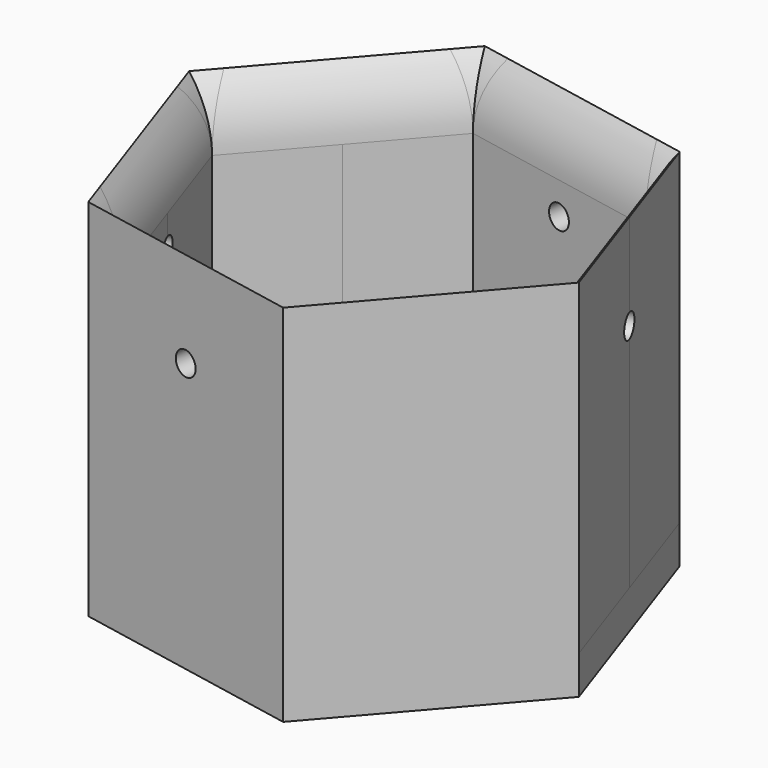
from build123d import *

# Parameters (mm, degrees)
F1_DEPTH      = 2.032
F3_DEPTH      = 19.05
F4_T4_DEPTH   = 36.3985226281
F4_T10_DEPTH  = 36.3985226281
F4_T16_DEPTH  = 36.3985226281
F4_T22_DEPTH  = 36.3985226281
F4_T28_DEPTH  = 36.3985226281
F4_T34_DEPTH  = 36.3985226281
F4_T41_DEPTH  = 36.3985226281
F4_T47_DEPTH  = 36.3985226281
F4_T56_DEPTH  = 36.3985226281
F4_T62_DEPTH  = 36.3985226281
F4_T71_DEPTH  = 36.3985226281
F4_T77_DEPTH  = 36.3985226281
F4_T86_DEPTH  = 36.3985226281
F4_T92_DEPTH  = 36.3985226281
F4_T101_DEPTH = 36.3985226281
F4_T107_DEPTH = 36.3985226281
F4_T116_DEPTH = 36.3985226281
F4_T122_DEPTH = 36.3985226281
F6_R          = 0.635
F7_DEPTH      = 25.4
F5_R          = 0.635
F8_DEPTH      = 25.4


# Not quite as in the source:
# - a fillet or chamfer that OpenCascade refuses, or shapes differently, is made with other operations: its cross-section is extruded or revolved along the edge and cut away or added


with BuildPart() as f1:
    # F0 (on Top) → F1 (new body)
    with BuildSketch(Plane.XY):
        Polygon((-123.0130245504, 41.1086249019), (-114.844562537, 50.5241579017), (-118.9144222983, 62.306020015), (-131.1527440729, 64.6723491286), (-139.3212060863, 55.2568161288), (-135.2513463251, 43.4749540155), align=None)
    extrude(amount=F1_DEPTH)

    # F2 (on face) → F3 (join)
    with BuildSketch(Plane.XY.offset(2.032)):
        Polygon((-131.1527440729, 64.6723491286), (-135.2369750796, 59.9645826287), (-134.2776702834, 59.1323360859), (-130.6739370422, 63.2862477035), (-119.8754178293, 61.1983102503), (-118.079891464, 56.0004299062), (-116.8794924177, 56.4150889583), (-118.9144222983, 62.306020015), align=None)
        Polygon((-134.2776702834, 59.1323360859), (-135.2369750796, 59.9645826287), (-139.3212060863, 55.2568161288), (-137.2862762057, 49.3658850722), (-136.0858771593, 49.7805441243), (-137.8814035246, 54.9784244684), align=None)
        Polygon((-136.0858771593, 49.7805441243), (-137.2862762057, 49.3658850722), (-135.2513463251, 43.4749540155), (-123.0130245504, 41.1086249019), (-118.9287935437, 45.8163914018), (-119.88809834, 46.6486379446), (-123.4918315812, 42.494726327), (-134.2903507941, 44.5826637802), align=None)
        Polygon((-116.2843650988, 50.8025495621), (-119.88809834, 46.6486379446), (-118.9287935437, 45.8163914018), (-114.844562537, 50.5241579017), (-116.8794924177, 56.4150889583), (-118.079891464, 56.0004299062), align=None)
    extrude(amount=F3_DEPTH)

    # F4: fillet of radius 5.08 on 6 edges, made by hand


with BuildPart() as f4_tool2:
    # F4_s3 → F4_t4 (new body)
    with BuildSketch(Plane(origin=(-40.3193780899, -46.4748975157, 0), x_dir=(0, 0, 1), z_dir=(0.6553122384, 0.7553581073, 0))):
        with BuildLine():
            ThreePointArc((21.082, -145.2578703952), (19.5941024484, -141.6657679468), (16.002, -140.1778703952))
            Line((16.002, -140.1778703952), (21.082, -140.1778703952))
            Line((21.082, -140.1778703952), (21.082, -145.2578703952))
        make_face()
    extrude(amount=F4_T4_DEPTH)

    split(bisect_by=Plane(origin=(7.0863744403, 36.6497331747, 0), x_dir=(0, 0, 1), z_dir=(-0.1898379922, -0.981815429, 0)), keep=Keep.TOP)

    split(bisect_by=Plane(origin=(-106.215781989, -36.6905785323, 0), x_dir=(0, 0, 1), z_dir=(0.9451960995, 0.3265031907, 0)), keep=Keep.TOP)


with BuildPart() as f1_1:
    add(f1.part)

    # F4_t1: cut F4_tool2
    add(f4_tool2.part, mode=Mode.SUBTRACT)


with BuildPart() as f4_tool8:
    # F4_s9 → F4_t10 (new body)
    with BuildSketch(Plane(origin=(-150.2293674314, 29.0474570301, 0), x_dir=(0, 0, 1), z_dir=(0.981815429, -0.1898379922, 0))):
        with BuildLine():
            ThreePointArc((21.082, -42.4085365971), (19.5941024484, -38.8164341487), (16.002, -37.3285365971))
            Line((16.002, -37.3285365971), (21.082, -37.3285365971))
            Line((21.082, -37.3285365971), (21.082, -42.4085365971))
        make_face()
    extrude(amount=F4_T10_DEPTH)

    split(bisect_by=Plane(origin=(-88.2097962936, -30.4706927504, 0), x_dir=(0, 0, 1), z_dir=(-0.9451960995, -0.3265031907, 0)), keep=Keep.TOP)

    split(bisect_by=Plane(origin=(-105.8844908623, 91.8602740219, 0), x_dir=(0, 0, 1), z_dir=(0.7553581073, -0.6553122384, 0)), keep=Keep.TOP)


with BuildPart() as f1_2:
    add(f1_1.part)

    # F4_t7: cut F4_tool8
    add(f4_tool8.part, mode=Mode.SUBTRACT)


with BuildPart() as f4_tool14:
    # F4_s15 → F4_t16 (new body)
    with BuildSketch(Plane(origin=(-35.8122120569, 103.6729934642, 0), x_dir=(0, 0, 1), z_dir=(0.3265031907, -0.9451960995, 0))):
        with BuildLine():
            ThreePointArc((21.082, 88.2443337981), (19.5941024484, 91.8364362465), (16.002, 93.3243337981))
            Line((16.002, 93.3243337981), (21.082, 93.3243337981))
            Line((21.082, 93.3243337981), (21.082, 88.2443337981))
        make_face()
    extrude(amount=F4_T16_DEPTH)

    split(bisect_by=Plane(origin=(-91.4949189189, 79.3765758805, 0), x_dir=(0, 0, 1), z_dir=(-0.7553581073, 0.6553122384, 0)), keep=Keep.TOP)

    split(bisect_by=Plane(origin=(7.0863744403, 36.6497331747, 0), x_dir=(0, 0, 1), z_dir=(-0.1898379922, -0.981815429, 0)), keep=Keep.TOP)


with BuildPart() as f1_3:
    add(f1_2.part)

    # F4_t13: cut F4_tool14
    add(f4_tool14.part, mode=Mode.SUBTRACT)


with BuildPart() as f4_tool20:
    # F4_s21 → F4_t22 (new body)
    with BuildSketch(Plane(origin=(-16.4669807523, -18.9809783561, 0), x_dir=(0, 0, 1), z_dir=(-0.6553122384, -0.7553581073, 0))):
        with BuildLine():
            ThreePointArc((21.082, 116.0478703952), (19.5941024484, 119.6399728436), (16.002, 121.1278703952))
            Line((16.002, 121.1278703952), (21.082, 121.1278703952))
            Line((21.082, 121.1278703952), (21.082, 116.0478703952))
        make_face()
    extrude(amount=F4_T22_DEPTH)

    split(bisect_by=Plane(origin=(-88.2097962936, -30.4706927504, 0), x_dir=(0, 0, 1), z_dir=(-0.9451960995, -0.3265031907, 0)), keep=Keep.TOP)

    split(bisect_by=Plane(origin=(3.4699606884, 17.9461492514, 0), x_dir=(0, 0, 1), z_dir=(0.1898379922, 0.981815429, 0)), keep=Keep.TOP)


with BuildPart() as f1_4:
    add(f1_3.part)

    # F4_t19: cut F4_tool20
    add(f4_tool20.part, mode=Mode.SUBTRACT)


with BuildPart() as f4_tool26:
    # F4_s27 → F4_t28 (new body)
    with BuildSketch(Plane(origin=(-114.4927363208, 22.1376345743, 0), x_dir=(0, 0, 1), z_dir=(-0.981815429, 0.1898379922, 0))):
        with BuildLine():
            ThreePointArc((21.082, 13.1985365971), (19.5941024484, 16.7906390456), (16.002, 18.2785365971))
            Line((16.002, 18.2785365971), (21.082, 18.2785365971))
            Line((21.082, 18.2785365971), (21.082, 13.1985365971))
        make_face()
    extrude(amount=F4_T28_DEPTH)

    split(bisect_by=Plane(origin=(-91.4949189189, 79.3765758805, 0), x_dir=(0, 0, 1), z_dir=(-0.7553581073, 0.6553122384, 0)), keep=Keep.TOP)

    split(bisect_by=Plane(origin=(-106.215781989, -36.6905785323, 0), x_dir=(0, 0, 1), z_dir=(0.9451960995, 0.3265031907, 0)), keep=Keep.TOP)


with BuildPart() as f1_5:
    add(f1_4.part)

    # F4_t25: cut F4_tool26
    add(f4_tool26.part, mode=Mode.SUBTRACT)


with BuildPart() as f4_tool32:
    # F4_s33 → F4_t34 (new body)
    with BuildSketch(Plane(origin=(-23.9279782839, 69.2692518489, 0), x_dir=(0, 0, 1), z_dir=(-0.3265031907, 0.9451960995, 0))):
        with BuildLine():
            ThreePointArc((21.082, -117.4543337981), (19.5941024484, -113.8622313496), (16.002, -112.3743337981))
            Line((16.002, -112.3743337981), (21.082, -112.3743337981))
            Line((21.082, -112.3743337981), (21.082, -117.4543337981))
        make_face()
    extrude(amount=F4_T34_DEPTH)

    split(bisect_by=Plane(origin=(-105.8844908623, 91.8602740219, 0), x_dir=(0, 0, 1), z_dir=(0.7553581073, -0.6553122384, 0)), keep=Keep.TOP)

    split(bisect_by=Plane(origin=(3.4699606884, 17.9461492514, 0), x_dir=(0, 0, 1), z_dir=(0.1898379922, 0.981815429, 0)), keep=Keep.TOP)


with BuildPart() as f1_6:
    add(f1_5.part)

    # F4_t31: cut F4_tool32
    add(f4_tool32.part, mode=Mode.SUBTRACT)


with BuildPart() as f4_tool39:
    # F4_s40 → F4_t41 (new body)
    with BuildSketch(Plane(origin=(-23.9279782839, 69.2692518489, 0), x_dir=(0, 0, 1), z_dir=(-0.3265031907, 0.9451960995, 0))):
        with BuildLine():
            ThreePointArc((21.082, -117.4543337981), (19.5941024484, -113.8622313496), (16.002, -112.3743337981))
            Line((16.002, -112.3743337981), (21.082, -112.3743337981))
            Line((21.082, -112.3743337981), (21.082, -117.4543337981))
        make_face()
    extrude(amount=F4_T41_DEPTH)

    split(bisect_by=Plane(origin=(-106.8437956585, 92.6925205646, 0), x_dir=(0, 0, 1), z_dir=(0.7553581073, -0.6553122384, 0)), keep=Keep.TOP)

    split(bisect_by=Plane(origin=(-105.8844908623, 91.8602740219, 0), x_dir=(0, 0, 1), z_dir=(-0.7553581073, 0.6553122384, 0)), keep=Keep.TOP)

    split(bisect_by=Plane(origin=(-107.4161810353, -37.1052375844, 0), x_dir=(0, 0, 1), z_dir=(0.9451960995, 0.3265031907, 0)), keep=Keep.TOP)


with BuildPart() as f4_tool45:
    # F4_s46 → F4_t47 (new body)
    with BuildSketch(Plane(origin=(-40.3193780899, -46.4748975157, 0), x_dir=(0, 0, 1), z_dir=(0.6553122384, 0.7553581073, 0))):
        with BuildLine():
            ThreePointArc((21.082, -145.2578703952), (19.5941024484, -141.6657679468), (16.002, -140.1778703952))
            Line((16.002, -140.1778703952), (21.082, -140.1778703952))
            Line((21.082, -140.1778703952), (21.082, -145.2578703952))
        make_face()
    extrude(amount=F4_T47_DEPTH)

    split(bisect_by=Plane(origin=(-106.8437956585, 92.6925205646, 0), x_dir=(0, 0, 1), z_dir=(0.7553581073, -0.6553122384, 0)), keep=Keep.TOP)

    split(bisect_by=Plane(origin=(-106.215781989, -36.6905785323, 0), x_dir=(0, 0, 1), z_dir=(-0.9451960995, -0.3265031907, 0)), keep=Keep.TOP)

    split(bisect_by=Plane(origin=(-107.4161810353, -37.1052375844, 0), x_dir=(0, 0, 1), z_dir=(0.9451960995, 0.3265031907, 0)), keep=Keep.TOP)


with BuildPart() as f4_tool39_1:
    add(f4_tool39.part)

    # F4_t51: intersect F4_tool45
    add(f4_tool45.part, mode=Mode.INTERSECT)


with BuildPart() as f1_7:
    add(f1_6.part)

    # F4_t37: cut F4_tool39
    add(f4_tool39_1.part, mode=Mode.SUBTRACT)


with BuildPart() as f4_tool54:
    # F4_s55 → F4_t56 (new body)
    with BuildSketch(Plane(origin=(-40.3193780899, -46.4748975157, 0), x_dir=(0, 0, 1), z_dir=(0.6553122384, 0.7553581073, 0))):
        with BuildLine():
            ThreePointArc((21.082, -145.2578703952), (19.5941024484, -141.6657679468), (16.002, -140.1778703952))
            Line((16.002, -140.1778703952), (21.082, -140.1778703952))
            Line((21.082, -140.1778703952), (21.082, -145.2578703952))
        make_face()
    extrude(amount=F4_T56_DEPTH)

    split(bisect_by=Plane(origin=(-106.8437956585, 92.6925205646, 0), x_dir=(0, 0, 1), z_dir=(0.7553581073, -0.6553122384, 0)), keep=Keep.TOP)

    split(bisect_by=Plane(origin=(7.3274686905, 37.8966387696, 0), x_dir=(0, 0, 1), z_dir=(-0.1898379922, -0.981815429, 0)), keep=Keep.TOP)

    split(bisect_by=Plane(origin=(7.0863744403, 36.6497331747, 0), x_dir=(0, 0, 1), z_dir=(0.1898379922, 0.981815429, 0)), keep=Keep.TOP)


with BuildPart() as f4_tool60:
    # F4_s61 → F4_t62 (new body)
    with BuildSketch(Plane(origin=(-150.2293674314, 29.0474570301, 0), x_dir=(0, 0, 1), z_dir=(0.981815429, -0.1898379922, 0))):
        with BuildLine():
            ThreePointArc((21.082, -42.4085365971), (19.5941024484, -38.8164341487), (16.002, -37.3285365971))
            Line((16.002, -37.3285365971), (21.082, -37.3285365971))
            Line((21.082, -37.3285365971), (21.082, -42.4085365971))
        make_face()
    extrude(amount=F4_T62_DEPTH)

    split(bisect_by=Plane(origin=(-106.8437956585, 92.6925205646, 0), x_dir=(0, 0, 1), z_dir=(0.7553581073, -0.6553122384, 0)), keep=Keep.TOP)

    split(bisect_by=Plane(origin=(7.3274686905, 37.8966387696, 0), x_dir=(0, 0, 1), z_dir=(-0.1898379922, -0.981815429, 0)), keep=Keep.TOP)

    split(bisect_by=Plane(origin=(-105.8844908623, 91.8602740219, 0), x_dir=(0, 0, 1), z_dir=(-0.7553581073, 0.6553122384, 0)), keep=Keep.TOP)


with BuildPart() as f4_tool54_1:
    add(f4_tool54.part)

    # F4_t66: intersect F4_tool60
    add(f4_tool60.part, mode=Mode.INTERSECT)


with BuildPart() as f1_8:
    add(f1_7.part)

    # F4_t52: cut F4_tool54
    add(f4_tool54_1.part, mode=Mode.SUBTRACT)


with BuildPart() as f4_tool69:
    # F4_s70 → F4_t71 (new body)
    with BuildSketch(Plane(origin=(-150.2293674314, 29.0474570301, 0), x_dir=(0, 0, 1), z_dir=(0.981815429, -0.1898379922, 0))):
        with BuildLine():
            ThreePointArc((21.082, -42.4085365971), (19.5941024484, -38.8164341487), (16.002, -37.3285365971))
            Line((16.002, -37.3285365971), (21.082, -37.3285365971))
            Line((21.082, -37.3285365971), (21.082, -42.4085365971))
        make_face()
    extrude(amount=F4_T71_DEPTH)

    split(bisect_by=Plane(origin=(7.3274686905, 37.8966387696, 0), x_dir=(0, 0, 1), z_dir=(-0.1898379922, -0.981815429, 0)), keep=Keep.TOP)

    split(bisect_by=Plane(origin=(-87.0093972473, -30.0560336983, 0), x_dir=(0, 0, 1), z_dir=(-0.9451960995, -0.3265031907, 0)), keep=Keep.TOP)

    split(bisect_by=Plane(origin=(-88.2097962936, -30.4706927504, 0), x_dir=(0, 0, 1), z_dir=(0.9451960995, 0.3265031907, 0)), keep=Keep.TOP)


with BuildPart() as f4_tool75:
    # F4_s76 → F4_t77 (new body)
    with BuildSketch(Plane(origin=(-35.8122120569, 103.6729934642, 0), x_dir=(0, 0, 1), z_dir=(0.3265031907, -0.9451960995, 0))):
        with BuildLine():
            ThreePointArc((21.082, 88.2443337981), (19.5941024484, 91.8364362465), (16.002, 93.3243337981))
            Line((16.002, 93.3243337981), (21.082, 93.3243337981))
            Line((21.082, 93.3243337981), (21.082, 88.2443337981))
        make_face()
    extrude(amount=F4_T77_DEPTH)

    split(bisect_by=Plane(origin=(7.3274686905, 37.8966387696, 0), x_dir=(0, 0, 1), z_dir=(-0.1898379922, -0.981815429, 0)), keep=Keep.TOP)

    split(bisect_by=Plane(origin=(-87.0093972473, -30.0560336983, 0), x_dir=(0, 0, 1), z_dir=(-0.9451960995, -0.3265031907, 0)), keep=Keep.TOP)

    split(bisect_by=Plane(origin=(7.0863744403, 36.6497331747, 0), x_dir=(0, 0, 1), z_dir=(0.1898379922, 0.981815429, 0)), keep=Keep.TOP)


with BuildPart() as f4_tool69_1:
    add(f4_tool69.part)

    # F4_t81: intersect F4_tool75
    add(f4_tool75.part, mode=Mode.INTERSECT)


with BuildPart() as f1_9:
    add(f1_8.part)

    # F4_t67: cut F4_tool69
    add(f4_tool69_1.part, mode=Mode.SUBTRACT)


with BuildPart() as f4_tool84:
    # F4_s85 → F4_t86 (new body)
    with BuildSketch(Plane(origin=(-35.8122120569, 103.6729934642, 0), x_dir=(0, 0, 1), z_dir=(0.3265031907, -0.9451960995, 0))):
        with BuildLine():
            ThreePointArc((21.082, 88.2443337981), (19.5941024484, 91.8364362465), (16.002, 93.3243337981))
            Line((16.002, 93.3243337981), (21.082, 93.3243337981))
            Line((21.082, 93.3243337981), (21.082, 88.2443337981))
        make_face()
    extrude(amount=F4_T86_DEPTH)

    split(bisect_by=Plane(origin=(-87.0093972473, -30.0560336983, 0), x_dir=(0, 0, 1), z_dir=(-0.9451960995, -0.3265031907, 0)), keep=Keep.TOP)

    split(bisect_by=Plane(origin=(-90.5356141227, 78.5443293377, 0), x_dir=(0, 0, 1), z_dir=(-0.7553581073, 0.6553122384, 0)), keep=Keep.TOP)

    split(bisect_by=Plane(origin=(-91.4949189189, 79.3765758805, 0), x_dir=(0, 0, 1), z_dir=(0.7553581073, -0.6553122384, 0)), keep=Keep.TOP)


with BuildPart() as f4_tool90:
    # F4_s91 → F4_t92 (new body)
    with BuildSketch(Plane(origin=(-16.4669807523, -18.9809783561, 0), x_dir=(0, 0, 1), z_dir=(-0.6553122384, -0.7553581073, 0))):
        with BuildLine():
            ThreePointArc((21.082, 116.0478703952), (19.5941024484, 119.6399728436), (16.002, 121.1278703952))
            Line((16.002, 121.1278703952), (21.082, 121.1278703952))
            Line((21.082, 121.1278703952), (21.082, 116.0478703952))
        make_face()
    extrude(amount=F4_T92_DEPTH)

    split(bisect_by=Plane(origin=(-87.0093972473, -30.0560336983, 0), x_dir=(0, 0, 1), z_dir=(-0.9451960995, -0.3265031907, 0)), keep=Keep.TOP)

    split(bisect_by=Plane(origin=(-90.5356141227, 78.5443293377, 0), x_dir=(0, 0, 1), z_dir=(-0.7553581073, 0.6553122384, 0)), keep=Keep.TOP)

    split(bisect_by=Plane(origin=(-88.2097962936, -30.4706927504, 0), x_dir=(0, 0, 1), z_dir=(0.9451960995, 0.3265031907, 0)), keep=Keep.TOP)


with BuildPart() as f4_tool84_1:
    add(f4_tool84.part)

    # F4_t96: intersect F4_tool90
    add(f4_tool90.part, mode=Mode.INTERSECT)


with BuildPart() as f1_10:
    add(f1_9.part)

    # F4_t82: cut F4_tool84
    add(f4_tool84_1.part, mode=Mode.SUBTRACT)


with BuildPart() as f4_tool99:
    # F4_s100 → F4_t101 (new body)
    with BuildSketch(Plane(origin=(-114.4927363208, 22.1376345743, 0), x_dir=(0, 0, 1), z_dir=(-0.981815429, 0.1898379922, 0))):
        with BuildLine():
            ThreePointArc((21.082, 13.1985365971), (19.5941024484, 16.7906390456), (16.002, 18.2785365971))
            Line((16.002, 18.2785365971), (21.082, 18.2785365971))
            Line((21.082, 18.2785365971), (21.082, 13.1985365971))
        make_face()
    extrude(amount=F4_T101_DEPTH)

    split(bisect_by=Plane(origin=(3.2288664383, 16.6992436565, 0), x_dir=(0, 0, 1), z_dir=(0.1898379922, 0.981815429, 0)), keep=Keep.TOP)

    split(bisect_by=Plane(origin=(-90.5356141227, 78.5443293377, 0), x_dir=(0, 0, 1), z_dir=(-0.7553581073, 0.6553122384, 0)), keep=Keep.TOP)

    split(bisect_by=Plane(origin=(-91.4949189189, 79.3765758805, 0), x_dir=(0, 0, 1), z_dir=(0.7553581073, -0.6553122384, 0)), keep=Keep.TOP)


with BuildPart() as f4_tool105:
    # F4_s106 → F4_t107 (new body)
    with BuildSketch(Plane(origin=(-16.4669807523, -18.9809783561, 0), x_dir=(0, 0, 1), z_dir=(-0.6553122384, -0.7553581073, 0))):
        with BuildLine():
            ThreePointArc((21.082, 116.0478703952), (19.5941024484, 119.6399728436), (16.002, 121.1278703952))
            Line((16.002, 121.1278703952), (21.082, 121.1278703952))
            Line((21.082, 121.1278703952), (21.082, 116.0478703952))
        make_face()
    extrude(amount=F4_T107_DEPTH)

    split(bisect_by=Plane(origin=(3.2288664383, 16.6992436565, 0), x_dir=(0, 0, 1), z_dir=(0.1898379922, 0.981815429, 0)), keep=Keep.TOP)

    split(bisect_by=Plane(origin=(-90.5356141227, 78.5443293377, 0), x_dir=(0, 0, 1), z_dir=(-0.7553581073, 0.6553122384, 0)), keep=Keep.TOP)

    split(bisect_by=Plane(origin=(3.4699606884, 17.9461492514, 0), x_dir=(0, 0, 1), z_dir=(-0.1898379922, -0.981815429, 0)), keep=Keep.TOP)


with BuildPart() as f4_tool99_1:
    add(f4_tool99.part)

    # F4_t111: intersect F4_tool105
    add(f4_tool105.part, mode=Mode.INTERSECT)


with BuildPart() as f1_11:
    add(f1_10.part)

    # F4_t97: cut F4_tool99
    add(f4_tool99_1.part, mode=Mode.SUBTRACT)


with BuildPart() as f4_tool114:
    # F4_s115 → F4_t116 (new body)
    with BuildSketch(Plane(origin=(-114.4927363208, 22.1376345743, 0), x_dir=(0, 0, 1), z_dir=(-0.981815429, 0.1898379922, 0))):
        with BuildLine():
            ThreePointArc((21.082, 13.1985365971), (19.5941024484, 16.7906390456), (16.002, 18.2785365971))
            Line((16.002, 18.2785365971), (21.082, 18.2785365971))
            Line((21.082, 18.2785365971), (21.082, 13.1985365971))
        make_face()
    extrude(amount=F4_T116_DEPTH)

    split(bisect_by=Plane(origin=(3.2288664383, 16.6992436565, 0), x_dir=(0, 0, 1), z_dir=(0.1898379922, 0.981815429, 0)), keep=Keep.TOP)

    split(bisect_by=Plane(origin=(-106.215781989, -36.6905785323, 0), x_dir=(0, 0, 1), z_dir=(-0.9451960995, -0.3265031907, 0)), keep=Keep.TOP)

    split(bisect_by=Plane(origin=(-107.4161810353, -37.1052375844, 0), x_dir=(0, 0, 1), z_dir=(0.9451960995, 0.3265031907, 0)), keep=Keep.TOP)


with BuildPart() as f4_tool120:
    # F4_s121 → F4_t122 (new body)
    with BuildSketch(Plane(origin=(-23.9279782839, 69.2692518489, 0), x_dir=(0, 0, 1), z_dir=(-0.3265031907, 0.9451960995, 0))):
        with BuildLine():
            ThreePointArc((21.082, -117.4543337981), (19.5941024484, -113.8622313496), (16.002, -112.3743337981))
            Line((16.002, -112.3743337981), (21.082, -112.3743337981))
            Line((21.082, -112.3743337981), (21.082, -117.4543337981))
        make_face()
    extrude(amount=F4_T122_DEPTH)

    split(bisect_by=Plane(origin=(3.2288664383, 16.6992436565, 0), x_dir=(0, 0, 1), z_dir=(0.1898379922, 0.981815429, 0)), keep=Keep.TOP)

    split(bisect_by=Plane(origin=(3.4699606884, 17.9461492514, 0), x_dir=(0, 0, 1), z_dir=(-0.1898379922, -0.981815429, 0)), keep=Keep.TOP)

    split(bisect_by=Plane(origin=(-107.4161810353, -37.1052375844, 0), x_dir=(0, 0, 1), z_dir=(0.9451960995, 0.3265031907, 0)), keep=Keep.TOP)


with BuildPart() as f4_tool114_1:
    add(f4_tool114.part)

    # F4_t126: intersect F4_tool120
    add(f4_tool120.part, mode=Mode.INTERSECT)


with BuildPart() as f1_12:
    add(f1_11.part)

    # F4_t112: cut F4_tool114
    add(f4_tool114_1.part, mode=Mode.SUBTRACT)

    # F6 (on face) → F7 (cut)
    with BuildSketch(Plane(origin=(7.3274686905, 37.8966387696, 0), x_dir=(-0.981815429, 0.1898379922, 0), z_dir=(0.1898379922, 0.981815429, 0))):
        with Locations((134.8125604474, 14.2821041651)):
            Circle(F6_R)
    extrude(amount=-F7_DEPTH, mode=Mode.SUBTRACT)

    # F5 (on face) → F8 (cut)
    with BuildSketch(Plane(origin=(-87.0093972473, -30.0560336983, 0), x_dir=(-0.3265031907, 0.9451960995, 0), z_dir=(0.9451960995, 0.3265031907, 0))):
        with Locations((91.4848492319, 14.2821041651)):
            Circle(F5_R)
    extrude(amount=-F8_DEPTH, mode=Mode.SUBTRACT)


solid = f1_12.part
